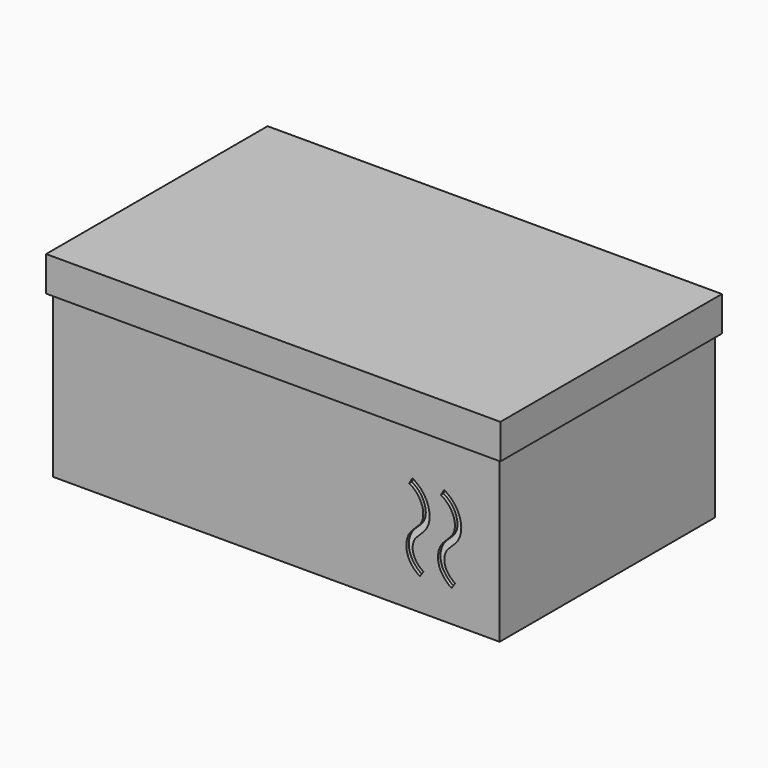
from build123d import *

# Parameters (mm, degrees)
F0_W     = 141
F0_H     = 85
F1_DEPTH = 51
F2_T     = -1
F4_DEPTH = 85
F5_W     = 143.4
F5_H     = 87.4
F5_W_2   = 141.4
F5_H_2   = 85.4
F6_DEPTH = 10
F7_W     = 143.4
F7_H     = 87.4
F8_DEPTH = 1


# Not quite as in the source:
# - the dataset's text gives a spline's control points without its knots; the knots are read off the source's solid


with BuildPart() as f1:
    # F0 (on Top) → F1 (new body)
    with BuildSketch(Plane.XY):
        Rectangle(F0_W, F0_H)
    extrude(amount=F1_DEPTH)

    # F2
    f2_openings = [f1.faces().sort_by_distance(p)[0] for p in [
        (0, 0, 51),
    ]]
    offset(amount=F2_T, openings=f2_openings)

    # F3 (on face) → F4 (cut, through all)
    with BuildSketch(Plane.XZ.offset(42.5)):
        with BuildLine():
            add(Edge.make_bspline(
                [(45.3295225173, 10), (40.5640363595, 13.175749098), (40.2028214903, 21.461601359), (47.9410200584, 24.8066902989), (45.9266969128, 32.5190219817), (41.9605416325, 34.786099143)],
                knots=[0, 0, 0, 0, 0.3682128641, 0.652025135, 1, 1, 1, 1], degree=3))
            Line((45.3295225173, 10), (46.4386226774, 11.6643007044))
            add(Edge.make_bspline(
                [(46.4386226774, 11.6643007044), (45.7540677896, 12.1204922651), (44.6487999007, 13.0778671585), (43.6301142093, 14.5512681872), (43.1079643944, 16.0118120012), (43.0068431553, 17.1867020343), (43.0921818636, 18.0655590198), (43.2300196743, 18.6814879329), (43.3969135453, 19.1469389206), (43.5551476766, 19.4843070413), (43.7252772316, 19.7928316255), (43.9784804349, 20.163479753), (44.353458668, 20.6073537767), (44.7986451103, 21.0638521449), (45.4728906234, 21.7070307175), (46.2420063611, 22.433622196), (47.0128954425, 23.3494461809), (47.4609979753, 24.0272596379), (47.7719295323, 24.6386230936), (47.974838358, 25.1344621316), (48.1358489655, 25.6469381667), (48.2972001691, 26.3457640196), (48.4031777442, 27.2451058164), (48.3794978137, 28.7215346751), (47.9966937541, 30.6094480092), (46.9607566355, 32.836760744), (45.3176808357, 34.8897247455), (43.8081956086, 36.0336475515), (42.9530514164, 36.5224528884)],
                knots=[0, 0, 0, 0, 0.0625, 0.125, 0.1875, 0.25, 0.28125, 0.3125, 0.34375, 0.359375, 0.375, 0.40625, 0.4375, 0.46875, 0.5, 0.5625, 0.59375, 0.625, 0.640625, 0.65625, 0.671875, 0.6875, 0.71875, 0.75, 0.8125, 0.875, 0.9375, 1, 1, 1, 1], degree=3))
            Line((42.9530514164, 36.5224528884), (41.9605416325, 34.786099143))
        make_face()
        with BuildLine():
            add(Edge.make_bspline(
                [(55.3295225173, 10), (50.5640363595, 13.175749098), (50.2028214903, 21.461601359), (57.9410200584, 24.8066902989), (55.9266969128, 32.5190219817), (51.9605416325, 34.786099143)],
                knots=[0, 0, 0, 0, 0.3682128641, 0.652025135, 1, 1, 1, 1], degree=3))
            Line((55.3295225173, 10), (56.4386226774, 11.6643007044))
            add(Edge.make_bspline(
                [(56.4386226774, 11.6643007044), (55.7540677896, 12.1204922651), (54.6487999007, 13.0778671585), (53.6301142093, 14.5512681872), (53.1079643944, 16.0118120012), (53.0068431553, 17.1867020343), (53.0921818636, 18.0655590198), (53.2300196743, 18.6814879329), (53.3969135453, 19.1469389206), (53.5551476766, 19.4843070413), (53.7252772316, 19.7928316255), (53.9784804349, 20.163479753), (54.353458668, 20.6073537767), (54.7986451103, 21.0638521449), (55.4728906234, 21.7070307175), (56.2420063611, 22.433622196), (57.0128954425, 23.3494461809), (57.4609979753, 24.0272596379), (57.7719295323, 24.6386230936), (57.974838358, 25.1344621316), (58.1358489655, 25.6469381667), (58.2972001691, 26.3457640196), (58.4031777442, 27.2451058164), (58.3794978137, 28.7215346751), (57.9966937541, 30.6094480092), (56.9607566355, 32.836760744), (55.3176808357, 34.8897247455), (53.8081956086, 36.0336475515), (52.9530514164, 36.5224528884)],
                knots=[0, 0, 0, 0, 0.0625, 0.125, 0.1875, 0.25, 0.28125, 0.3125, 0.34375, 0.359375, 0.375, 0.40625, 0.4375, 0.46875, 0.5, 0.5625, 0.59375, 0.625, 0.640625, 0.65625, 0.671875, 0.6875, 0.71875, 0.75, 0.8125, 0.875, 0.9375, 1, 1, 1, 1], degree=3))
            Line((52.9530514164, 36.5224528884), (51.9605416325, 34.786099143))
        make_face()
    extrude(amount=-F4_DEPTH, mode=Mode.SUBTRACT)


with BuildPart() as f6:
    # F5 (on face) → F6 (new body)
    with BuildSketch(Plane.XY.offset(51)):
        Rectangle(F5_W, F5_H)
        Rectangle(F5_W_2, F5_H_2, mode=Mode.SUBTRACT)
    extrude(amount=F6_DEPTH)

    # F7 (on face) → F8 (join)
    with BuildSketch(Plane.XY.offset(61)):
        Rectangle(F7_W, F7_H)
    extrude(amount=F8_DEPTH)


solid = Compound([f1.part, f6.part])
